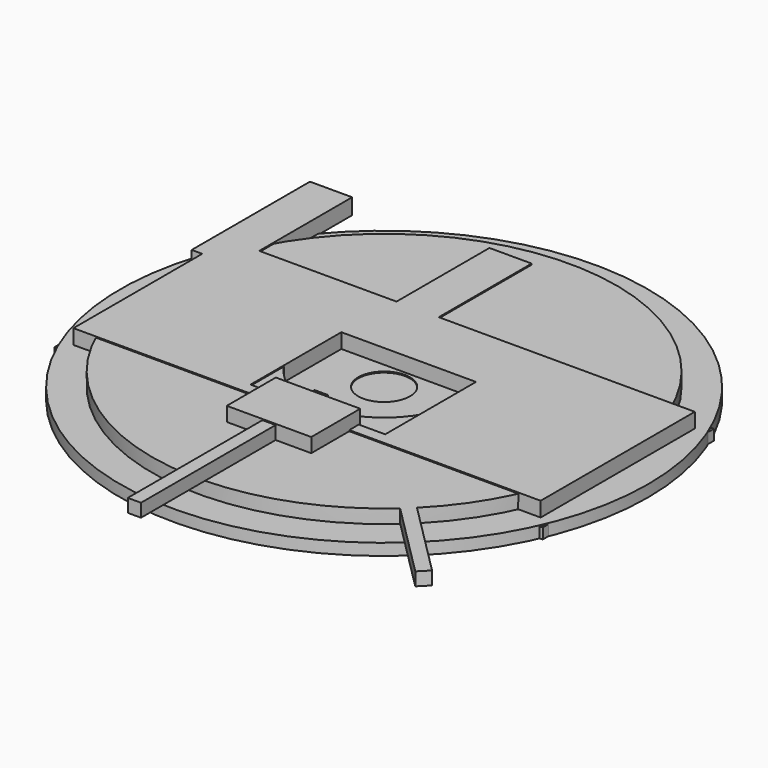
from build123d import *

# Parameters (mm, degrees)
F0_R      = 0.875
F1_DEPTH  = 1
F2_W      = 12.75
F2_H      = 10.75
F3_DEPTH  = 1.5
F4_W      = 8
F4_H      = 5.8
F5_DEPTH  = 2.75
F6_W      = 4
F6_H      = 1.5
F7_DEPTH  = 10
F8_R      = 25
F8_R_2    = 2.45
F9_DEPTH  = 1.1
F10_R     = 22
F10_R_2   = 7.45
F11_DEPTH = 1.3
F13_DEPTH = 1.25
F14_DEPTH = 1.25


with BuildPart() as f1:
    # F0 (on Top) → F1 (new body)
    with BuildSketch(Plane.XY):
        Polygon((23.125, 10.125), (-23.125, 10.125), (-23.125, -10.125), (-6, -10.125), (-6, -12.125), (6, -12.125), (6, -10.125), (23.125, -10.125), align=None)
        with Locations((-4.375, -6.125)):
            Circle(F0_R, mode=Mode.SUBTRACT)
        with Locations((4.625, 0.875)):
            Circle(F0_R, mode=Mode.SUBTRACT)
    extrude(amount=F1_DEPTH)

    # F2 (on face) → F3 (join)
    with BuildSketch(Plane.XY.offset(1)):
        Polygon((-6.125, 9.125), (-19.125, 9.125), (-19.125, 10.125), (-23.125, 10.125), (-23.125, 6.125), (-22.125, 6.125), (-22.125, -9.125), (22.125, -9.125), (22.125, 9.125), (-2.125, 9.125), (-2.125, 10.125), (-6.125, 10.125), align=None)
        with Locations((0.125, -2.625)):
            Rectangle(F2_W, F2_H, mode=Mode.SUBTRACT)
    extrude(amount=F3_DEPTH)

    # F4 (on face) → F5 (join)
    with BuildSketch(Plane.XY.offset(1)):
        with Locations((0, -10.725)):
            Rectangle(F4_W, F4_H)
    extrude(amount=F5_DEPTH)

    # F6 (on face) → F7 (join)
    with BuildSketch(Plane(origin=(0, 10.125, 0), x_dir=(-1, 0, 0), z_dir=(0, 1, 0))):
        with Locations((4.125, 1.75)):
            Rectangle(F6_W, F6_H)
        with Locations((21.125, 1.75)):
            Rectangle(F6_W, F6_H)
    extrude(amount=F7_DEPTH)


with BuildPart() as f9:
    # F8 (on Top) → F9 (new body)
    with BuildSketch(Plane.XY):
        Circle(F8_R)
        Circle(F8_R_2, mode=Mode.SUBTRACT)
    extrude(amount=F9_DEPTH)

    # F10 (on face) → F11 (join)
    with BuildSketch(Plane.XY.offset(1.1)):
        Circle(F10_R)
        Circle(F10_R_2, mode=Mode.SUBTRACT)
    extrude(amount=F11_DEPTH)

    # F12 (on face) → F13 (join)
    with BuildSketch(Plane.XY.offset(2.4)):
        with BuildLine():
            Line((0, -7.45), (-0.625, -7.45))
            Line((-0.625, -7.45), (-0.625, -21.9911203671))
            ThreePointArc((-0.625, -21.9911203671), (0, -22), (0.625, -21.9911203671))
            Line((0.625, -21.9911203671), (0.625, -7.45))
            Line((0.625, -7.45), (0, -7.45))
        make_face()
        with BuildLine():
            ThreePointArc((0.625, -21.9911203671), (0, -22), (-0.625, -21.9911203671))
            Line((-0.625, -21.9911203671), (-0.625, -29.5649133623))
            Line((-0.625, -29.5649133623), (0.625, -29.5649133623))
            Line((0.625, -29.5649133623), (0.625, -21.9911203671))
        make_face()
    extrude(amount=F13_DEPTH)

    # F12 (on face) → F14 (join)
    with BuildSketch(Plane.XY.offset(2.4)):
        with BuildLine():
            ThreePointArc((14.6473350849, -16.4151020378), (15.1079449297, -15.9921855917), (15.5563491861, -15.5563491861))
            Line((15.5563491861, -15.5563491861), (14.8492424049, -14.8492424049))
            Line((14.8492424049, -14.8492424049), (13.9653589284, -15.7331258814))
            Line((13.9653589284, -15.7331258814), (14.6473350849, -16.4151020378))
        make_face()
        with BuildLine():
            Line((22.7137225264, -22.7137225264), (15.5563491861, -15.5563491861))
            ThreePointArc((15.5563491861, -15.5563491861), (15.1079449297, -15.9921855917), (14.6473350849, -16.4151020378))
            Line((14.6473350849, -16.4151020378), (21.8298390499, -23.5976060029))
            Line((21.8298390499, -23.5976060029), (22.7137225264, -22.7137225264))
        make_face()
    extrude(amount=-F14_DEPTH)


solid = Compound([f1.part, f9.part])
